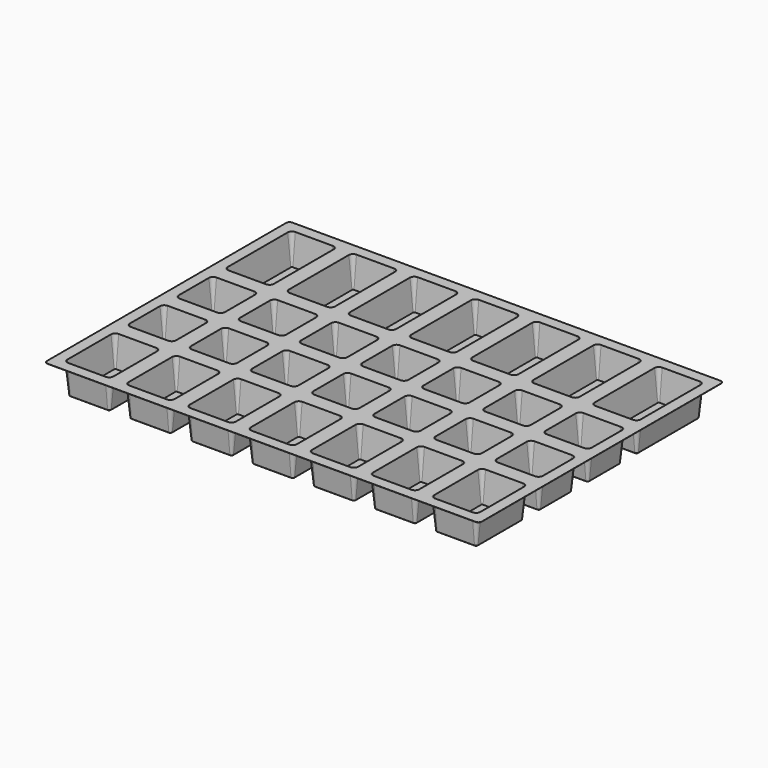
from build123d import *

# Parameters (mm, degrees)
F1_W     = 256
F1_H     = 180
F2_DEPTH = 0.1
F3_DEPTH = 25
F4_DEPTH = 18
F4_TAPER = 6
F5_T     = 0.5
F5_2_T   = -0.5
F5_3_T   = 0.5
F5_4_T   = 0.5
F5_5_T   = -0.5
F5_6_T   = 0.5
F5_7_T   = 0.5
F5_8_T   = -0.5
F5_9_T   = -0.5
F5_10_T  = 0.5
F5_11_T  = 0.5
F5_12_T  = -0.5
F5_13_T  = -0.5
F5_14_T  = 0.5
F5_15_T  = 0.5
F5_16_T  = -0.5
F5_17_T  = -0.5
F5_18_T  = 0.5
F5_19_T  = -0.5
F5_20_T  = 0.5
F5_21_T  = 0.5
F5_22_T  = -0.5
F5_23_T  = 0.5
F5_24_T  = -0.5
F5_25_T  = -0.5
F5_26_T  = 0.5
F5_27_T  = -0.5
F5_28_T  = 0.5
F6_R     = 2
F7_R     = 0.5
F7_2_R   = 0.5
F7_3_R   = 0.5
F7_4_R   = 0.5
F7_5_R   = 0.5
F7_6_R   = 0.5
F7_7_R   = 0.5
F7_8_R   = 0.5
F7_9_R   = 0.5
F7_10_R  = 0.5
F7_11_R  = 0.5
F7_12_R  = 0.5
F7_13_R  = 0.5
F7_14_R  = 0.5
F7_15_R  = 0.5
F7_16_R  = 0.5
F7_17_R  = 0.5
F7_18_R  = 0.5
F7_19_R  = 0.5
F7_20_R  = 0.5
F7_21_R  = 0.5
F7_22_R  = 0.5
F7_23_R  = 0.5
F7_24_R  = 0.5
F7_25_R  = 0.5
F7_26_R  = 0.5
F7_27_R  = 0.5
F7_28_R  = 0.5


# Not quite as in the source:
# - a shell that OpenCascade refuses in one call is made with other operations: the cavity is built on its own and cut out


with BuildPart() as f2:
    # F1 (on Top) → F2 (new body)
    with BuildSketch(Plane.XY):
        with Locations((132.6459416151, -90)):
            Rectangle(F1_W, F1_H)
    extrude(amount=-F2_DEPTH)

    # F0 (on Top) → F3 (cut)
    with BuildSketch(Plane.XY):
        with BuildLine():
            ThreePointArc((121.6459416151, -6), (119.5246212715, -6.8786796564), (118.6459416151, -9))
            Line((118.6459416151, -9), (118.6459416151, -53))
            ThreePointArc((118.6459416151, -53), (119.5246212715, -55.1213203436), (121.6459416151, -56))
            Line((121.6459416151, -56), (143.6459416151, -56))
            ThreePointArc((143.6459416151, -56), (145.7672619587, -55.1213203436), (146.6459416151, -53))
            Line((146.6459416151, -53), (146.6459416151, -9))
            ThreePointArc((146.6459416151, -9), (145.7672619587, -6.8786796564), (143.6459416151, -6))
            Line((143.6459416151, -6), (121.6459416151, -6))
        make_face()
        with BuildLine():
            Line((146.6459416151, -89), (146.6459416151, -67))
            ThreePointArc((146.6459416151, -67), (145.7672619587, -64.8786796564), (143.6459416151, -64))
            Line((143.6459416151, -64), (121.6459416151, -64))
            ThreePointArc((121.6459416151, -64), (119.5246212715, -64.8786796564), (118.6459416151, -67))
            Line((118.6459416151, -67), (118.6459416151, -89))
            ThreePointArc((118.6459416151, -89), (119.5246212715, -91.1213203436), (121.6459416151, -92))
            Line((121.6459416151, -92), (143.6459416151, -92))
            ThreePointArc((143.6459416151, -92), (145.7672619587, -91.1213203436), (146.6459416151, -89))
        make_face()
        with BuildLine():
            Line((146.6459416151, -125), (146.6459416151, -103))
            ThreePointArc((146.6459416151, -103), (145.7672619587, -100.8786796564), (143.6459416151, -100))
            Line((143.6459416151, -100), (121.6459416151, -100))
            ThreePointArc((121.6459416151, -100), (119.5246212715, -100.8786796564), (118.6459416151, -103))
            Line((118.6459416151, -103), (118.6459416151, -125))
            ThreePointArc((118.6459416151, -125), (119.5246212715, -127.1213203436), (121.6459416151, -128))
            Line((121.6459416151, -128), (143.6459416151, -128))
            ThreePointArc((143.6459416151, -128), (145.7672619587, -127.1213203436), (146.6459416151, -125))
        make_face()
        with BuildLine():
            Line((146.6459416151, -171), (146.6459416151, -139))
            ThreePointArc((146.6459416151, -139), (145.7672619587, -136.8786796564), (143.6459416151, -136))
            Line((143.6459416151, -136), (121.6459416151, -136))
            ThreePointArc((121.6459416151, -136), (119.5246212715, -136.8786796564), (118.6459416151, -139))
            Line((118.6459416151, -139), (118.6459416151, -171))
            ThreePointArc((118.6459416151, -171), (119.5246212715, -173.1213203436), (121.6459416151, -174))
            Line((121.6459416151, -174), (143.6459416151, -174))
            ThreePointArc((143.6459416151, -174), (145.7672619587, -173.1213203436), (146.6459416151, -171))
        make_face()
        with BuildLine():
            ThreePointArc((157.6459416151, -6), (155.5246212715, -6.8786796564), (154.6459416151, -9))
            Line((154.6459416151, -9), (154.6459416151, -53))
            ThreePointArc((154.6459416151, -53), (155.5246212715, -55.1213203436), (157.6459416151, -56))
            Line((157.6459416151, -56), (179.6459416151, -56))
            ThreePointArc((179.6459416151, -56), (181.7672619587, -55.1213203436), (182.6459416151, -53))
            Line((182.6459416151, -53), (182.6459416151, -9))
            ThreePointArc((182.6459416151, -9), (181.7672619587, -6.8786796564), (179.6459416151, -6))
            Line((179.6459416151, -6), (157.6459416151, -6))
        make_face()
        with BuildLine():
            Line((182.6459416151, -89), (182.6459416151, -67))
            ThreePointArc((182.6459416151, -67), (181.7672619587, -64.8786796564), (179.6459416151, -64))
            Line((179.6459416151, -64), (157.6459416151, -64))
            ThreePointArc((157.6459416151, -64), (155.5246212715, -64.8786796564), (154.6459416151, -67))
            Line((154.6459416151, -67), (154.6459416151, -89))
            ThreePointArc((154.6459416151, -89), (155.5246212715, -91.1213203436), (157.6459416151, -92))
            Line((157.6459416151, -92), (179.6459416151, -92))
            ThreePointArc((179.6459416151, -92), (181.7672619587, -91.1213203436), (182.6459416151, -89))
        make_face()
        with BuildLine():
            ThreePointArc((157.6459416151, -136), (155.5246212715, -136.8786796564), (154.6459416151, -139))
            Line((154.6459416151, -139), (154.6459416151, -171))
            ThreePointArc((154.6459416151, -171), (155.5246212715, -173.1213203436), (157.6459416151, -174))
            Line((157.6459416151, -174), (179.6459416151, -174))
            ThreePointArc((179.6459416151, -174), (181.7672619587, -173.1213203436), (182.6459416151, -171))
            Line((182.6459416151, -171), (182.6459416151, -139))
            ThreePointArc((182.6459416151, -139), (181.7672619587, -136.8786796564), (179.6459416151, -136))
            Line((179.6459416151, -136), (157.6459416151, -136))
        make_face()
        with BuildLine():
            Line((182.6459416151, -125), (182.6459416151, -103))
            ThreePointArc((182.6459416151, -103), (181.7672619587, -100.8786796564), (179.6459416151, -100))
            Line((179.6459416151, -100), (157.6459416151, -100))
            ThreePointArc((157.6459416151, -100), (155.5246212715, -100.8786796564), (154.6459416151, -103))
            Line((154.6459416151, -103), (154.6459416151, -125))
            ThreePointArc((154.6459416151, -125), (155.5246212715, -127.1213203436), (157.6459416151, -128))
            Line((157.6459416151, -128), (179.6459416151, -128))
            ThreePointArc((179.6459416151, -128), (181.7672619587, -127.1213203436), (182.6459416151, -125))
        make_face()
        with BuildLine():
            ThreePointArc((193.6459416151, -6), (191.5246212715, -6.8786796564), (190.6459416151, -9))
            Line((190.6459416151, -9), (190.6459416151, -53))
            ThreePointArc((190.6459416151, -53), (191.5246212715, -55.1213203436), (193.6459416151, -56))
            Line((193.6459416151, -56), (215.6459416151, -56))
            ThreePointArc((215.6459416151, -56), (217.7672619587, -55.1213203436), (218.6459416151, -53))
            Line((218.6459416151, -53), (218.6459416151, -9))
            ThreePointArc((218.6459416151, -9), (217.7672619587, -6.8786796564), (215.6459416151, -6))
            Line((215.6459416151, -6), (193.6459416151, -6))
        make_face()
        with BuildLine():
            Line((218.6459416151, -89), (218.6459416151, -67))
            ThreePointArc((218.6459416151, -67), (217.7672619587, -64.8786796564), (215.6459416151, -64))
            Line((215.6459416151, -64), (193.6459416151, -64))
            ThreePointArc((193.6459416151, -64), (191.5246212715, -64.8786796564), (190.6459416151, -67))
            Line((190.6459416151, -67), (190.6459416151, -89))
            ThreePointArc((190.6459416151, -89), (191.5246212715, -91.1213203436), (193.6459416151, -92))
            Line((193.6459416151, -92), (215.6459416151, -92))
            ThreePointArc((215.6459416151, -92), (217.7672619587, -91.1213203436), (218.6459416151, -89))
        make_face()
        with BuildLine():
            ThreePointArc((193.6459416151, -136), (191.5246212715, -136.8786796564), (190.6459416151, -139))
            Line((190.6459416151, -139), (190.6459416151, -171))
            ThreePointArc((190.6459416151, -171), (191.5246212715, -173.1213203436), (193.6459416151, -174))
            Line((193.6459416151, -174), (215.6459416151, -174))
            ThreePointArc((215.6459416151, -174), (217.7672619587, -173.1213203436), (218.6459416151, -171))
            Line((218.6459416151, -171), (218.6459416151, -139))
            ThreePointArc((218.6459416151, -139), (217.7672619587, -136.8786796564), (215.6459416151, -136))
            Line((215.6459416151, -136), (193.6459416151, -136))
        make_face()
        with BuildLine():
            Line((218.6459416151, -125), (218.6459416151, -103))
            ThreePointArc((218.6459416151, -103), (217.7672619587, -100.8786796564), (215.6459416151, -100))
            Line((215.6459416151, -100), (193.6459416151, -100))
            ThreePointArc((193.6459416151, -100), (191.5246212715, -100.8786796564), (190.6459416151, -103))
            Line((190.6459416151, -103), (190.6459416151, -125))
            ThreePointArc((190.6459416151, -125), (191.5246212715, -127.1213203436), (193.6459416151, -128))
            Line((193.6459416151, -128), (215.6459416151, -128))
            ThreePointArc((215.6459416151, -128), (217.7672619587, -127.1213203436), (218.6459416151, -125))
        make_face()
        with BuildLine():
            ThreePointArc((229.6459416151, -6), (227.5246212715, -6.8786796564), (226.6459416151, -9))
            Line((226.6459416151, -9), (226.6459416151, -53))
            ThreePointArc((226.6459416151, -53), (227.5246212715, -55.1213203436), (229.6459416151, -56))
            Line((229.6459416151, -56), (251.6459416151, -56))
            ThreePointArc((251.6459416151, -56), (253.7672619587, -55.1213203436), (254.6459416151, -53))
            Line((254.6459416151, -53), (254.6459416151, -9))
            ThreePointArc((254.6459416151, -9), (253.7672619587, -6.8786796564), (251.6459416151, -6))
            Line((251.6459416151, -6), (229.6459416151, -6))
        make_face()
        with BuildLine():
            Line((254.6459416151, -89), (254.6459416151, -67))
            ThreePointArc((254.6459416151, -67), (253.7672619587, -64.8786796564), (251.6459416151, -64))
            Line((251.6459416151, -64), (229.6459416151, -64))
            ThreePointArc((229.6459416151, -64), (227.5246212715, -64.8786796564), (226.6459416151, -67))
            Line((226.6459416151, -67), (226.6459416151, -89))
            ThreePointArc((226.6459416151, -89), (227.5246212715, -91.1213203436), (229.6459416151, -92))
            Line((229.6459416151, -92), (251.6459416151, -92))
            ThreePointArc((251.6459416151, -92), (253.7672619587, -91.1213203436), (254.6459416151, -89))
        make_face()
        with BuildLine():
            ThreePointArc((229.6459416151, -136), (227.5246212715, -136.8786796564), (226.6459416151, -139))
            Line((226.6459416151, -139), (226.6459416151, -171))
            ThreePointArc((226.6459416151, -171), (227.5246212715, -173.1213203436), (229.6459416151, -174))
            Line((229.6459416151, -174), (251.6459416151, -174))
            ThreePointArc((251.6459416151, -174), (253.7672619587, -173.1213203436), (254.6459416151, -171))
            Line((254.6459416151, -171), (254.6459416151, -139))
            ThreePointArc((254.6459416151, -139), (253.7672619587, -136.8786796564), (251.6459416151, -136))
            Line((251.6459416151, -136), (229.6459416151, -136))
        make_face()
        with BuildLine():
            Line((254.6459416151, -125), (254.6459416151, -103))
            ThreePointArc((254.6459416151, -103), (253.7672619587, -100.8786796564), (251.6459416151, -100))
            Line((251.6459416151, -100), (229.6459416151, -100))
            ThreePointArc((229.6459416151, -100), (227.5246212715, -100.8786796564), (226.6459416151, -103))
            Line((226.6459416151, -103), (226.6459416151, -125))
            ThreePointArc((226.6459416151, -125), (227.5246212715, -127.1213203436), (229.6459416151, -128))
            Line((229.6459416151, -128), (251.6459416151, -128))
            ThreePointArc((251.6459416151, -128), (253.7672619587, -127.1213203436), (254.6459416151, -125))
        make_face()
        with BuildLine():
            Line((85.6459416151, -92), (107.6459416151, -92))
            ThreePointArc((107.6459416151, -92), (109.7672619587, -91.1213203436), (110.6459416151, -89))
            Line((110.6459416151, -89), (110.6459416151, -67))
            ThreePointArc((110.6459416151, -67), (109.7672619587, -64.8786796564), (107.6459416151, -64))
            Line((107.6459416151, -64), (85.6459416151, -64))
            ThreePointArc((85.6459416151, -64), (83.5246212715, -64.8786796564), (82.6459416151, -67))
            Line((82.6459416151, -67), (82.6459416151, -89))
            ThreePointArc((82.6459416151, -89), (83.5246212715, -91.1213203436), (85.6459416151, -92))
        make_face()
        with BuildLine():
            Line((85.6459416151, -128), (107.6459416151, -128))
            ThreePointArc((107.6459416151, -128), (109.7672619587, -127.1213203436), (110.6459416151, -125))
            Line((110.6459416151, -125), (110.6459416151, -103))
            ThreePointArc((110.6459416151, -103), (109.7672619587, -100.8786796564), (107.6459416151, -100))
            Line((107.6459416151, -100), (85.6459416151, -100))
            ThreePointArc((85.6459416151, -100), (83.5246212715, -100.8786796564), (82.6459416151, -103))
            Line((82.6459416151, -103), (82.6459416151, -125))
            ThreePointArc((82.6459416151, -125), (83.5246212715, -127.1213203436), (85.6459416151, -128))
        make_face()
        with BuildLine():
            ThreePointArc((85.6459416151, -136), (83.5246212715, -136.8786796564), (82.6459416151, -139))
            Line((82.6459416151, -139), (82.6459416151, -171))
            ThreePointArc((82.6459416151, -171), (83.5246212715, -173.1213203436), (85.6459416151, -174))
            Line((85.6459416151, -174), (107.6459416151, -174))
            ThreePointArc((107.6459416151, -174), (109.7672619587, -173.1213203436), (110.6459416151, -171))
            Line((110.6459416151, -171), (110.6459416151, -139))
            ThreePointArc((110.6459416151, -139), (109.7672619587, -136.8786796564), (107.6459416151, -136))
            Line((107.6459416151, -136), (85.6459416151, -136))
        make_face()
        with BuildLine():
            Line((110.6459416151, -53), (110.6459416151, -9))
            ThreePointArc((110.6459416151, -9), (109.7672619587, -6.8786796564), (107.6459416151, -6))
            Line((107.6459416151, -6), (85.6459416151, -6))
            ThreePointArc((85.6459416151, -6), (83.5246212715, -6.8786796564), (82.6459416151, -9))
            Line((82.6459416151, -9), (82.6459416151, -53))
            ThreePointArc((82.6459416151, -53), (83.5246212715, -55.1213203436), (85.6459416151, -56))
            Line((85.6459416151, -56), (107.6459416151, -56))
            ThreePointArc((107.6459416151, -56), (109.7672619587, -55.1213203436), (110.6459416151, -53))
        make_face()
        with BuildLine():
            Line((49.6459416151, -92), (71.6459416151, -92))
            ThreePointArc((71.6459416151, -92), (73.7672619587, -91.1213203436), (74.6459416151, -89))
            Line((74.6459416151, -89), (74.6459416151, -67))
            ThreePointArc((74.6459416151, -67), (73.7672619587, -64.8786796564), (71.6459416151, -64))
            Line((71.6459416151, -64), (49.6459416151, -64))
            ThreePointArc((49.6459416151, -64), (47.5246212715, -64.8786796564), (46.6459416151, -67))
            Line((46.6459416151, -67), (46.6459416151, -89))
            ThreePointArc((46.6459416151, -89), (47.5246212715, -91.1213203436), (49.6459416151, -92))
        make_face()
        with BuildLine():
            Line((49.6459416151, -128), (71.6459416151, -128))
            ThreePointArc((71.6459416151, -128), (73.7672619587, -127.1213203436), (74.6459416151, -125))
            Line((74.6459416151, -125), (74.6459416151, -103))
            ThreePointArc((74.6459416151, -103), (73.7672619587, -100.8786796564), (71.6459416151, -100))
            Line((71.6459416151, -100), (49.6459416151, -100))
            ThreePointArc((49.6459416151, -100), (47.5246212715, -100.8786796564), (46.6459416151, -103))
            Line((46.6459416151, -103), (46.6459416151, -125))
            ThreePointArc((46.6459416151, -125), (47.5246212715, -127.1213203436), (49.6459416151, -128))
        make_face()
        with BuildLine():
            ThreePointArc((49.6459416151, -136), (47.5246212715, -136.8786796564), (46.6459416151, -139))
            Line((46.6459416151, -139), (46.6459416151, -171))
            ThreePointArc((46.6459416151, -171), (47.5246212715, -173.1213203436), (49.6459416151, -174))
            Line((49.6459416151, -174), (71.6459416151, -174))
            ThreePointArc((71.6459416151, -174), (73.7672619587, -173.1213203436), (74.6459416151, -171))
            Line((74.6459416151, -171), (74.6459416151, -139))
            ThreePointArc((74.6459416151, -139), (73.7672619587, -136.8786796564), (71.6459416151, -136))
            Line((71.6459416151, -136), (49.6459416151, -136))
        make_face()
        with BuildLine():
            Line((74.6459416151, -53), (74.6459416151, -9))
            ThreePointArc((74.6459416151, -9), (73.7672619587, -6.8786796564), (71.6459416151, -6))
            Line((71.6459416151, -6), (49.6459416151, -6))
            ThreePointArc((49.6459416151, -6), (47.5246212715, -6.8786796564), (46.6459416151, -9))
            Line((46.6459416151, -9), (46.6459416151, -53))
            ThreePointArc((46.6459416151, -53), (47.5246212715, -55.1213203436), (49.6459416151, -56))
            Line((49.6459416151, -56), (71.6459416151, -56))
            ThreePointArc((71.6459416151, -56), (73.7672619587, -55.1213203436), (74.6459416151, -53))
        make_face()
        with BuildLine():
            Line((13.6459416151, -92), (35.6459416151, -92))
            ThreePointArc((35.6459416151, -92), (37.7672619587, -91.1213203436), (38.6459416151, -89))
            Line((38.6459416151, -89), (38.6459416151, -67))
            ThreePointArc((38.6459416151, -67), (37.7672619587, -64.8786796564), (35.6459416151, -64))
            Line((35.6459416151, -64), (13.6459416151, -64))
            ThreePointArc((13.6459416151, -64), (11.5246212715, -64.8786796564), (10.6459416151, -67))
            Line((10.6459416151, -67), (10.6459416151, -89))
            ThreePointArc((10.6459416151, -89), (11.5246212715, -91.1213203436), (13.6459416151, -92))
        make_face()
        with BuildLine():
            Line((13.6459416151, -128), (35.6459416151, -128))
            ThreePointArc((35.6459416151, -128), (37.7672619587, -127.1213203436), (38.6459416151, -125))
            Line((38.6459416151, -125), (38.6459416151, -103))
            ThreePointArc((38.6459416151, -103), (37.7672619587, -100.8786796564), (35.6459416151, -100))
            Line((35.6459416151, -100), (13.6459416151, -100))
            ThreePointArc((13.6459416151, -100), (11.5246212715, -100.8786796564), (10.6459416151, -103))
            Line((10.6459416151, -103), (10.6459416151, -125))
            ThreePointArc((10.6459416151, -125), (11.5246212715, -127.1213203436), (13.6459416151, -128))
        make_face()
        with BuildLine():
            ThreePointArc((13.6459416151, -136), (11.5246212715, -136.8786796564), (10.6459416151, -139))
            Line((10.6459416151, -139), (10.6459416151, -171))
            ThreePointArc((10.6459416151, -171), (11.5246212715, -173.1213203436), (13.6459416151, -174))
            Line((13.6459416151, -174), (35.6459416151, -174))
            ThreePointArc((35.6459416151, -174), (37.7672619587, -173.1213203436), (38.6459416151, -171))
            Line((38.6459416151, -171), (38.6459416151, -139))
            ThreePointArc((38.6459416151, -139), (37.7672619587, -136.8786796564), (35.6459416151, -136))
            Line((35.6459416151, -136), (13.6459416151, -136))
        make_face()
        with BuildLine():
            Line((38.6459416151, -53), (38.6459416151, -9))
            ThreePointArc((38.6459416151, -9), (37.7672619587, -6.8786796564), (35.6459416151, -6))
            Line((35.6459416151, -6), (13.6459416151, -6))
            ThreePointArc((13.6459416151, -6), (11.5246212715, -6.8786796564), (10.6459416151, -9))
            Line((10.6459416151, -9), (10.6459416151, -53))
            ThreePointArc((10.6459416151, -53), (11.5246212715, -55.1213203436), (13.6459416151, -56))
            Line((13.6459416151, -56), (35.6459416151, -56))
            ThreePointArc((35.6459416151, -56), (37.7672619587, -55.1213203436), (38.6459416151, -53))
        make_face()
    extrude(amount=-F3_DEPTH, mode=Mode.SUBTRACT)

    # F6
    f6_edges = [f2.edges().sort_by_distance(p)[0] for p in [
        (4.645942, -180, -0.05),
        (260.645942, -180, -0.05),
        (260.645942, 0, -0.05),
        (4.645942, 0, -0.05),
    ]]
    fillet(f6_edges, radius=F6_R)


with BuildPart() as f4:
    # F0 (on Top) → F4 (new body)
    with BuildSketch(Plane.XY):
        with BuildLine():
            ThreePointArc((121.6459416151, -6), (119.5246212715, -6.8786796564), (118.6459416151, -9))
            Line((118.6459416151, -9), (118.6459416151, -53))
            ThreePointArc((118.6459416151, -53), (119.5246212715, -55.1213203436), (121.6459416151, -56))
            Line((121.6459416151, -56), (143.6459416151, -56))
            ThreePointArc((143.6459416151, -56), (145.7672619587, -55.1213203436), (146.6459416151, -53))
            Line((146.6459416151, -53), (146.6459416151, -9))
            ThreePointArc((146.6459416151, -9), (145.7672619587, -6.8786796564), (143.6459416151, -6))
            Line((143.6459416151, -6), (121.6459416151, -6))
        make_face()
    extrude(amount=-F4_DEPTH, taper=F4_TAPER)

    # F5: shell of thickness 0.5, made by hand


with BuildPart() as f4b:
    # F0 (on Top) → F4, piece 2 (new body)
    with BuildSketch(Plane.XY):
        with BuildLine():
            Line((146.6459416151, -89), (146.6459416151, -67))
            ThreePointArc((146.6459416151, -67), (145.7672619587, -64.8786796564), (143.6459416151, -64))
            Line((143.6459416151, -64), (121.6459416151, -64))
            ThreePointArc((121.6459416151, -64), (119.5246212715, -64.8786796564), (118.6459416151, -67))
            Line((118.6459416151, -67), (118.6459416151, -89))
            ThreePointArc((118.6459416151, -89), (119.5246212715, -91.1213203436), (121.6459416151, -92))
            Line((121.6459416151, -92), (143.6459416151, -92))
            ThreePointArc((143.6459416151, -92), (145.7672619587, -91.1213203436), (146.6459416151, -89))
        make_face()
    extrude(amount=-F4_DEPTH, taper=F4_TAPER)

    # F5#2
    f5_2_openings = [f4b.faces().sort_by_distance(p)[0] for p in [
        (132.645942, -78, 0),
    ]]
    offset(amount=F5_2_T, openings=f5_2_openings)

    # F7#2
    f7_2_edges = [f4b.edges().sort_by_distance(p)[0] for p in [
        (144.429503, -89.783562, -18),
        (144.754065, -78, -18),
        (144.429503, -66.216438, -18),
        (132.645942, -65.891876, -18),
        (120.86238, -66.216438, -18),
        (120.537818, -78, -18),
        (120.86238, -89.783562, -18),
        (132.645942, -90.108124, -18),
    ]]
    fillet(f7_2_edges, radius=F7_2_R)


with BuildPart() as f4c:
    # F0 (on Top) → F4, piece 3 (new body)
    with BuildSketch(Plane.XY):
        with BuildLine():
            Line((146.6459416151, -125), (146.6459416151, -103))
            ThreePointArc((146.6459416151, -103), (145.7672619587, -100.8786796564), (143.6459416151, -100))
            Line((143.6459416151, -100), (121.6459416151, -100))
            ThreePointArc((121.6459416151, -100), (119.5246212715, -100.8786796564), (118.6459416151, -103))
            Line((118.6459416151, -103), (118.6459416151, -125))
            ThreePointArc((118.6459416151, -125), (119.5246212715, -127.1213203436), (121.6459416151, -128))
            Line((121.6459416151, -128), (143.6459416151, -128))
            ThreePointArc((143.6459416151, -128), (145.7672619587, -127.1213203436), (146.6459416151, -125))
        make_face()
    extrude(amount=-F4_DEPTH, taper=F4_TAPER)

    # F5#3: shell of thickness 0.5, made by hand


with BuildPart() as f4d:
    # F0 (on Top) → F4, piece 4 (new body)
    with BuildSketch(Plane.XY):
        with BuildLine():
            Line((146.6459416151, -171), (146.6459416151, -139))
            ThreePointArc((146.6459416151, -139), (145.7672619587, -136.8786796564), (143.6459416151, -136))
            Line((143.6459416151, -136), (121.6459416151, -136))
            ThreePointArc((121.6459416151, -136), (119.5246212715, -136.8786796564), (118.6459416151, -139))
            Line((118.6459416151, -139), (118.6459416151, -171))
            ThreePointArc((118.6459416151, -171), (119.5246212715, -173.1213203436), (121.6459416151, -174))
            Line((121.6459416151, -174), (143.6459416151, -174))
            ThreePointArc((143.6459416151, -174), (145.7672619587, -173.1213203436), (146.6459416151, -171))
        make_face()
    extrude(amount=-F4_DEPTH, taper=F4_TAPER)

    # F5#4: shell of thickness 0.5, made by hand


with BuildPart() as f4e:
    # F0 (on Top) → F4, piece 5 (new body)
    with BuildSketch(Plane.XY):
        with BuildLine():
            ThreePointArc((157.6459416151, -6), (155.5246212715, -6.8786796564), (154.6459416151, -9))
            Line((154.6459416151, -9), (154.6459416151, -53))
            ThreePointArc((154.6459416151, -53), (155.5246212715, -55.1213203436), (157.6459416151, -56))
            Line((157.6459416151, -56), (179.6459416151, -56))
            ThreePointArc((179.6459416151, -56), (181.7672619587, -55.1213203436), (182.6459416151, -53))
            Line((182.6459416151, -53), (182.6459416151, -9))
            ThreePointArc((182.6459416151, -9), (181.7672619587, -6.8786796564), (179.6459416151, -6))
            Line((179.6459416151, -6), (157.6459416151, -6))
        make_face()
    extrude(amount=-F4_DEPTH, taper=F4_TAPER)

    # F5#13
    f5_13_openings = [f4e.faces().sort_by_distance(p)[0] for p in [
        (168.645942, -31, 0),
    ]]
    offset(amount=F5_13_T, openings=f5_13_openings)

    # F7#17
    f7_17_edges = [f4e.edges().sort_by_distance(p)[0] for p in [
        (156.86238, -8.216438, -18),
        (156.537818, -31, -18),
        (156.86238, -53.783562, -18),
        (168.645942, -54.108124, -18),
        (180.429503, -53.783562, -18),
        (180.754065, -31, -18),
        (180.429503, -8.216438, -18),
        (168.645942, -7.891876, -18),
    ]]
    fillet(f7_17_edges, radius=F7_17_R)


with BuildPart() as f4f:
    # F0 (on Top) → F4, piece 6 (new body)
    with BuildSketch(Plane.XY):
        with BuildLine():
            Line((182.6459416151, -89), (182.6459416151, -67))
            ThreePointArc((182.6459416151, -67), (181.7672619587, -64.8786796564), (179.6459416151, -64))
            Line((179.6459416151, -64), (157.6459416151, -64))
            ThreePointArc((157.6459416151, -64), (155.5246212715, -64.8786796564), (154.6459416151, -67))
            Line((154.6459416151, -67), (154.6459416151, -89))
            ThreePointArc((154.6459416151, -89), (155.5246212715, -91.1213203436), (157.6459416151, -92))
            Line((157.6459416151, -92), (179.6459416151, -92))
            ThreePointArc((179.6459416151, -92), (181.7672619587, -91.1213203436), (182.6459416151, -89))
        make_face()
    extrude(amount=-F4_DEPTH, taper=F4_TAPER)

    # F5#14: shell of thickness 0.5, made by hand


with BuildPart() as f4g:
    # F0 (on Top) → F4, piece 7 (new body)
    with BuildSketch(Plane.XY):
        with BuildLine():
            ThreePointArc((157.6459416151, -136), (155.5246212715, -136.8786796564), (154.6459416151, -139))
            Line((154.6459416151, -139), (154.6459416151, -171))
            ThreePointArc((154.6459416151, -171), (155.5246212715, -173.1213203436), (157.6459416151, -174))
            Line((157.6459416151, -174), (179.6459416151, -174))
            ThreePointArc((179.6459416151, -174), (181.7672619587, -173.1213203436), (182.6459416151, -171))
            Line((182.6459416151, -171), (182.6459416151, -139))
            ThreePointArc((182.6459416151, -139), (181.7672619587, -136.8786796564), (179.6459416151, -136))
            Line((179.6459416151, -136), (157.6459416151, -136))
        make_face()
    extrude(amount=-F4_DEPTH, taper=F4_TAPER)

    # F5#16
    f5_16_openings = [f4g.faces().sort_by_distance(p)[0] for p in [
        (168.645942, -155, 0),
    ]]
    offset(amount=F5_16_T, openings=f5_16_openings)

    # F7#20
    f7_20_edges = [f4g.edges().sort_by_distance(p)[0] for p in [
        (180.429503, -138.216438, -18),
        (168.645942, -137.891876, -18),
        (156.86238, -138.216438, -18),
        (156.537818, -155, -18),
        (156.86238, -171.783562, -18),
        (168.645942, -172.108124, -18),
        (180.429503, -171.783562, -18),
        (180.754065, -155, -18),
    ]]
    fillet(f7_20_edges, radius=F7_20_R)


with BuildPart() as f4h:
    # F0 (on Top) → F4, piece 8 (new body)
    with BuildSketch(Plane.XY):
        with BuildLine():
            Line((182.6459416151, -125), (182.6459416151, -103))
            ThreePointArc((182.6459416151, -103), (181.7672619587, -100.8786796564), (179.6459416151, -100))
            Line((179.6459416151, -100), (157.6459416151, -100))
            ThreePointArc((157.6459416151, -100), (155.5246212715, -100.8786796564), (154.6459416151, -103))
            Line((154.6459416151, -103), (154.6459416151, -125))
            ThreePointArc((154.6459416151, -125), (155.5246212715, -127.1213203436), (157.6459416151, -128))
            Line((157.6459416151, -128), (179.6459416151, -128))
            ThreePointArc((179.6459416151, -128), (181.7672619587, -127.1213203436), (182.6459416151, -125))
        make_face()
    extrude(amount=-F4_DEPTH, taper=F4_TAPER)

    # F5#15: shell of thickness 0.5, made by hand


with BuildPart() as f4i:
    # F0 (on Top) → F4, piece 9 (new body)
    with BuildSketch(Plane.XY):
        with BuildLine():
            ThreePointArc((193.6459416151, -6), (191.5246212715, -6.8786796564), (190.6459416151, -9))
            Line((190.6459416151, -9), (190.6459416151, -53))
            ThreePointArc((190.6459416151, -53), (191.5246212715, -55.1213203436), (193.6459416151, -56))
            Line((193.6459416151, -56), (215.6459416151, -56))
            ThreePointArc((215.6459416151, -56), (217.7672619587, -55.1213203436), (218.6459416151, -53))
            Line((218.6459416151, -53), (218.6459416151, -9))
            ThreePointArc((218.6459416151, -9), (217.7672619587, -6.8786796564), (215.6459416151, -6))
            Line((215.6459416151, -6), (193.6459416151, -6))
        make_face()
    extrude(amount=-F4_DEPTH, taper=F4_TAPER)

    # F5#12
    f5_12_openings = [f4i.faces().sort_by_distance(p)[0] for p in [
        (204.645942, -31, 0),
    ]]
    offset(amount=F5_12_T, openings=f5_12_openings)

    # F7#24
    f7_24_edges = [f4i.edges().sort_by_distance(p)[0] for p in [
        (192.86238, -8.216438, -18),
        (192.537818, -31, -18),
        (192.86238, -53.783562, -18),
        (204.645942, -54.108124, -18),
        (216.429503, -53.783562, -18),
        (216.754065, -31, -18),
        (216.429503, -8.216438, -18),
        (204.645942, -7.891876, -18),
    ]]
    fillet(f7_24_edges, radius=F7_24_R)


with BuildPart() as f4j:
    # F0 (on Top) → F4, piece 10 (new body)
    with BuildSketch(Plane.XY):
        with BuildLine():
            Line((218.6459416151, -89), (218.6459416151, -67))
            ThreePointArc((218.6459416151, -67), (217.7672619587, -64.8786796564), (215.6459416151, -64))
            Line((215.6459416151, -64), (193.6459416151, -64))
            ThreePointArc((193.6459416151, -64), (191.5246212715, -64.8786796564), (190.6459416151, -67))
            Line((190.6459416151, -67), (190.6459416151, -89))
            ThreePointArc((190.6459416151, -89), (191.5246212715, -91.1213203436), (193.6459416151, -92))
            Line((193.6459416151, -92), (215.6459416151, -92))
            ThreePointArc((215.6459416151, -92), (217.7672619587, -91.1213203436), (218.6459416151, -89))
        make_face()
    extrude(amount=-F4_DEPTH, taper=F4_TAPER)

    # F5#11: shell of thickness 0.5, made by hand


with BuildPart() as f4k:
    # F0 (on Top) → F4, piece 11 (new body)
    with BuildSketch(Plane.XY):
        with BuildLine():
            ThreePointArc((193.6459416151, -136), (191.5246212715, -136.8786796564), (190.6459416151, -139))
            Line((190.6459416151, -139), (190.6459416151, -171))
            ThreePointArc((190.6459416151, -171), (191.5246212715, -173.1213203436), (193.6459416151, -174))
            Line((193.6459416151, -174), (215.6459416151, -174))
            ThreePointArc((215.6459416151, -174), (217.7672619587, -173.1213203436), (218.6459416151, -171))
            Line((218.6459416151, -171), (218.6459416151, -139))
            ThreePointArc((218.6459416151, -139), (217.7672619587, -136.8786796564), (215.6459416151, -136))
            Line((215.6459416151, -136), (193.6459416151, -136))
        make_face()
    extrude(amount=-F4_DEPTH, taper=F4_TAPER)

    # F5#9
    f5_9_openings = [f4k.faces().sort_by_distance(p)[0] for p in [
        (204.645942, -155, 0),
    ]]
    offset(amount=F5_9_T, openings=f5_9_openings)

    # F7#21
    f7_21_edges = [f4k.edges().sort_by_distance(p)[0] for p in [
        (216.429503, -138.216438, -18),
        (204.645942, -137.891876, -18),
        (192.86238, -138.216438, -18),
        (192.537818, -155, -18),
        (192.86238, -171.783562, -18),
        (204.645942, -172.108124, -18),
        (216.429503, -171.783562, -18),
        (216.754065, -155, -18),
    ]]
    fillet(f7_21_edges, radius=F7_21_R)


with BuildPart() as f4l:
    # F0 (on Top) → F4, piece 12 (new body)
    with BuildSketch(Plane.XY):
        with BuildLine():
            Line((218.6459416151, -125), (218.6459416151, -103))
            ThreePointArc((218.6459416151, -103), (217.7672619587, -100.8786796564), (215.6459416151, -100))
            Line((215.6459416151, -100), (193.6459416151, -100))
            ThreePointArc((193.6459416151, -100), (191.5246212715, -100.8786796564), (190.6459416151, -103))
            Line((190.6459416151, -103), (190.6459416151, -125))
            ThreePointArc((190.6459416151, -125), (191.5246212715, -127.1213203436), (193.6459416151, -128))
            Line((193.6459416151, -128), (215.6459416151, -128))
            ThreePointArc((215.6459416151, -128), (217.7672619587, -127.1213203436), (218.6459416151, -125))
        make_face()
    extrude(amount=-F4_DEPTH, taper=F4_TAPER)

    # F5#10: shell of thickness 0.5, made by hand


with BuildPart() as f4m:
    # F0 (on Top) → F4, piece 13 (new body)
    with BuildSketch(Plane.XY):
        with BuildLine():
            ThreePointArc((229.6459416151, -6), (227.5246212715, -6.8786796564), (226.6459416151, -9))
            Line((226.6459416151, -9), (226.6459416151, -53))
            ThreePointArc((226.6459416151, -53), (227.5246212715, -55.1213203436), (229.6459416151, -56))
            Line((229.6459416151, -56), (251.6459416151, -56))
            ThreePointArc((251.6459416151, -56), (253.7672619587, -55.1213203436), (254.6459416151, -53))
            Line((254.6459416151, -53), (254.6459416151, -9))
            ThreePointArc((254.6459416151, -9), (253.7672619587, -6.8786796564), (251.6459416151, -6))
            Line((251.6459416151, -6), (229.6459416151, -6))
        make_face()
    extrude(amount=-F4_DEPTH, taper=F4_TAPER)

    # F5#5
    f5_5_openings = [f4m.faces().sort_by_distance(p)[0] for p in [
        (240.645942, -31, 0),
    ]]
    offset(amount=F5_5_T, openings=f5_5_openings)

    # F7#25
    f7_25_edges = [f4m.edges().sort_by_distance(p)[0] for p in [
        (228.86238, -8.216438, -18),
        (228.537818, -31, -18),
        (228.86238, -53.783562, -18),
        (240.645942, -54.108124, -18),
        (252.429503, -53.783562, -18),
        (252.754065, -31, -18),
        (252.429503, -8.216438, -18),
        (240.645942, -7.891876, -18),
    ]]
    fillet(f7_25_edges, radius=F7_25_R)


with BuildPart() as f4n:
    # F0 (on Top) → F4, piece 14 (new body)
    with BuildSketch(Plane.XY):
        with BuildLine():
            Line((254.6459416151, -89), (254.6459416151, -67))
            ThreePointArc((254.6459416151, -67), (253.7672619587, -64.8786796564), (251.6459416151, -64))
            Line((251.6459416151, -64), (229.6459416151, -64))
            ThreePointArc((229.6459416151, -64), (227.5246212715, -64.8786796564), (226.6459416151, -67))
            Line((226.6459416151, -67), (226.6459416151, -89))
            ThreePointArc((226.6459416151, -89), (227.5246212715, -91.1213203436), (229.6459416151, -92))
            Line((229.6459416151, -92), (251.6459416151, -92))
            ThreePointArc((251.6459416151, -92), (253.7672619587, -91.1213203436), (254.6459416151, -89))
        make_face()
    extrude(amount=-F4_DEPTH, taper=F4_TAPER)

    # F5#6: shell of thickness 0.5, made by hand


with BuildPart() as f4o:
    # F0 (on Top) → F4, piece 15 (new body)
    with BuildSketch(Plane.XY):
        with BuildLine():
            ThreePointArc((229.6459416151, -136), (227.5246212715, -136.8786796564), (226.6459416151, -139))
            Line((226.6459416151, -139), (226.6459416151, -171))
            ThreePointArc((226.6459416151, -171), (227.5246212715, -173.1213203436), (229.6459416151, -174))
            Line((229.6459416151, -174), (251.6459416151, -174))
            ThreePointArc((251.6459416151, -174), (253.7672619587, -173.1213203436), (254.6459416151, -171))
            Line((254.6459416151, -171), (254.6459416151, -139))
            ThreePointArc((254.6459416151, -139), (253.7672619587, -136.8786796564), (251.6459416151, -136))
            Line((251.6459416151, -136), (229.6459416151, -136))
        make_face()
    extrude(amount=-F4_DEPTH, taper=F4_TAPER)

    # F5#8
    f5_8_openings = [f4o.faces().sort_by_distance(p)[0] for p in [
        (240.645942, -155, 0),
    ]]
    offset(amount=F5_8_T, openings=f5_8_openings)

    # F7#28
    f7_28_edges = [f4o.edges().sort_by_distance(p)[0] for p in [
        (252.429503, -138.216438, -18),
        (240.645942, -137.891876, -18),
        (228.86238, -138.216438, -18),
        (228.537818, -155, -18),
        (228.86238, -171.783562, -18),
        (240.645942, -172.108124, -18),
        (252.429503, -171.783562, -18),
        (252.754065, -155, -18),
    ]]
    fillet(f7_28_edges, radius=F7_28_R)


with BuildPart() as f4p:
    # F0 (on Top) → F4, piece 16 (new body)
    with BuildSketch(Plane.XY):
        with BuildLine():
            Line((254.6459416151, -125), (254.6459416151, -103))
            ThreePointArc((254.6459416151, -103), (253.7672619587, -100.8786796564), (251.6459416151, -100))
            Line((251.6459416151, -100), (229.6459416151, -100))
            ThreePointArc((229.6459416151, -100), (227.5246212715, -100.8786796564), (226.6459416151, -103))
            Line((226.6459416151, -103), (226.6459416151, -125))
            ThreePointArc((226.6459416151, -125), (227.5246212715, -127.1213203436), (229.6459416151, -128))
            Line((229.6459416151, -128), (251.6459416151, -128))
            ThreePointArc((251.6459416151, -128), (253.7672619587, -127.1213203436), (254.6459416151, -125))
        make_face()
    extrude(amount=-F4_DEPTH, taper=F4_TAPER)

    # F5#7: shell of thickness 0.5, made by hand


with BuildPart() as f4q:
    # F0 (on Top) → F4, piece 17 (new body)
    with BuildSketch(Plane.XY):
        with BuildLine():
            Line((85.6459416151, -92), (107.6459416151, -92))
            ThreePointArc((107.6459416151, -92), (109.7672619587, -91.1213203436), (110.6459416151, -89))
            Line((110.6459416151, -89), (110.6459416151, -67))
            ThreePointArc((110.6459416151, -67), (109.7672619587, -64.8786796564), (107.6459416151, -64))
            Line((107.6459416151, -64), (85.6459416151, -64))
            ThreePointArc((85.6459416151, -64), (83.5246212715, -64.8786796564), (82.6459416151, -67))
            Line((82.6459416151, -67), (82.6459416151, -89))
            ThreePointArc((82.6459416151, -89), (83.5246212715, -91.1213203436), (85.6459416151, -92))
        make_face()
    extrude(amount=-F4_DEPTH, taper=F4_TAPER)

    # F5#19
    f5_19_openings = [f4q.faces().sort_by_distance(p)[0] for p in [
        (96.645942, -78, 0),
    ]]
    offset(amount=F5_19_T, openings=f5_19_openings)

    # F7#15
    f7_15_edges = [f4q.edges().sort_by_distance(p)[0] for p in [
        (84.86238, -89.783562, -18),
        (96.645942, -90.108124, -18),
        (108.429503, -89.783562, -18),
        (108.754065, -78, -18),
        (108.429503, -66.216438, -18),
        (96.645942, -65.891876, -18),
        (84.86238, -66.216438, -18),
        (84.537818, -78, -18),
    ]]
    fillet(f7_15_edges, radius=F7_15_R)


with BuildPart() as f4r:
    # F0 (on Top) → F4, piece 18 (new body)
    with BuildSketch(Plane.XY):
        with BuildLine():
            Line((85.6459416151, -128), (107.6459416151, -128))
            ThreePointArc((107.6459416151, -128), (109.7672619587, -127.1213203436), (110.6459416151, -125))
            Line((110.6459416151, -125), (110.6459416151, -103))
            ThreePointArc((110.6459416151, -103), (109.7672619587, -100.8786796564), (107.6459416151, -100))
            Line((107.6459416151, -100), (85.6459416151, -100))
            ThreePointArc((85.6459416151, -100), (83.5246212715, -100.8786796564), (82.6459416151, -103))
            Line((82.6459416151, -103), (82.6459416151, -125))
            ThreePointArc((82.6459416151, -125), (83.5246212715, -127.1213203436), (85.6459416151, -128))
        make_face()
    extrude(amount=-F4_DEPTH, taper=F4_TAPER)

    # F5#18: shell of thickness 0.5, made by hand


with BuildPart() as f4s:
    # F0 (on Top) → F4, piece 19 (new body)
    with BuildSketch(Plane.XY):
        with BuildLine():
            ThreePointArc((85.6459416151, -136), (83.5246212715, -136.8786796564), (82.6459416151, -139))
            Line((82.6459416151, -139), (82.6459416151, -171))
            ThreePointArc((82.6459416151, -171), (83.5246212715, -173.1213203436), (85.6459416151, -174))
            Line((85.6459416151, -174), (107.6459416151, -174))
            ThreePointArc((107.6459416151, -174), (109.7672619587, -173.1213203436), (110.6459416151, -171))
            Line((110.6459416151, -171), (110.6459416151, -139))
            ThreePointArc((110.6459416151, -139), (109.7672619587, -136.8786796564), (107.6459416151, -136))
            Line((107.6459416151, -136), (85.6459416151, -136))
        make_face()
    extrude(amount=-F4_DEPTH, taper=F4_TAPER)

    # F5#17
    f5_17_openings = [f4s.faces().sort_by_distance(p)[0] for p in [
        (96.645942, -155, 0),
    ]]
    offset(amount=F5_17_T, openings=f5_17_openings)

    # F7#13
    f7_13_edges = [f4s.edges().sort_by_distance(p)[0] for p in [
        (108.429503, -138.216438, -18),
        (96.645942, -137.891876, -18),
        (84.86238, -138.216438, -18),
        (84.537818, -155, -18),
        (84.86238, -171.783562, -18),
        (96.645942, -172.108124, -18),
        (108.429503, -171.783562, -18),
        (108.754065, -155, -18),
    ]]
    fillet(f7_13_edges, radius=F7_13_R)


with BuildPart() as f4t:
    # F0 (on Top) → F4, piece 20 (new body)
    with BuildSketch(Plane.XY):
        with BuildLine():
            Line((110.6459416151, -53), (110.6459416151, -9))
            ThreePointArc((110.6459416151, -9), (109.7672619587, -6.8786796564), (107.6459416151, -6))
            Line((107.6459416151, -6), (85.6459416151, -6))
            ThreePointArc((85.6459416151, -6), (83.5246212715, -6.8786796564), (82.6459416151, -9))
            Line((82.6459416151, -9), (82.6459416151, -53))
            ThreePointArc((82.6459416151, -53), (83.5246212715, -55.1213203436), (85.6459416151, -56))
            Line((85.6459416151, -56), (107.6459416151, -56))
            ThreePointArc((107.6459416151, -56), (109.7672619587, -55.1213203436), (110.6459416151, -53))
        make_face()
    extrude(amount=-F4_DEPTH, taper=F4_TAPER)

    # F5#20: shell of thickness 0.5, made by hand


with BuildPart() as f4u:
    # F0 (on Top) → F4, piece 21 (new body)
    with BuildSketch(Plane.XY):
        with BuildLine():
            Line((49.6459416151, -92), (71.6459416151, -92))
            ThreePointArc((71.6459416151, -92), (73.7672619587, -91.1213203436), (74.6459416151, -89))
            Line((74.6459416151, -89), (74.6459416151, -67))
            ThreePointArc((74.6459416151, -67), (73.7672619587, -64.8786796564), (71.6459416151, -64))
            Line((71.6459416151, -64), (49.6459416151, -64))
            ThreePointArc((49.6459416151, -64), (47.5246212715, -64.8786796564), (46.6459416151, -67))
            Line((46.6459416151, -67), (46.6459416151, -89))
            ThreePointArc((46.6459416151, -89), (47.5246212715, -91.1213203436), (49.6459416151, -92))
        make_face()
    extrude(amount=-F4_DEPTH, taper=F4_TAPER)

    # F5#22
    f5_22_openings = [f4u.faces().sort_by_distance(p)[0] for p in [
        (60.645942, -78, 0),
    ]]
    offset(amount=F5_22_T, openings=f5_22_openings)

    # F7#10
    f7_10_edges = [f4u.edges().sort_by_distance(p)[0] for p in [
        (48.86238, -89.783562, -18),
        (60.645942, -90.108124, -18),
        (72.429503, -89.783562, -18),
        (72.754065, -78, -18),
        (72.429503, -66.216438, -18),
        (60.645942, -65.891876, -18),
        (48.86238, -66.216438, -18),
        (48.537818, -78, -18),
    ]]
    fillet(f7_10_edges, radius=F7_10_R)


with BuildPart() as f4v:
    # F0 (on Top) → F4, piece 22 (new body)
    with BuildSketch(Plane.XY):
        with BuildLine():
            Line((49.6459416151, -128), (71.6459416151, -128))
            ThreePointArc((71.6459416151, -128), (73.7672619587, -127.1213203436), (74.6459416151, -125))
            Line((74.6459416151, -125), (74.6459416151, -103))
            ThreePointArc((74.6459416151, -103), (73.7672619587, -100.8786796564), (71.6459416151, -100))
            Line((71.6459416151, -100), (49.6459416151, -100))
            ThreePointArc((49.6459416151, -100), (47.5246212715, -100.8786796564), (46.6459416151, -103))
            Line((46.6459416151, -103), (46.6459416151, -125))
            ThreePointArc((46.6459416151, -125), (47.5246212715, -127.1213203436), (49.6459416151, -128))
        make_face()
    extrude(amount=-F4_DEPTH, taper=F4_TAPER)

    # F5#23: shell of thickness 0.5, made by hand


with BuildPart() as f4w:
    # F0 (on Top) → F4, piece 23 (new body)
    with BuildSketch(Plane.XY):
        with BuildLine():
            ThreePointArc((49.6459416151, -136), (47.5246212715, -136.8786796564), (46.6459416151, -139))
            Line((46.6459416151, -139), (46.6459416151, -171))
            ThreePointArc((46.6459416151, -171), (47.5246212715, -173.1213203436), (49.6459416151, -174))
            Line((49.6459416151, -174), (71.6459416151, -174))
            ThreePointArc((71.6459416151, -174), (73.7672619587, -173.1213203436), (74.6459416151, -171))
            Line((74.6459416151, -171), (74.6459416151, -139))
            ThreePointArc((74.6459416151, -139), (73.7672619587, -136.8786796564), (71.6459416151, -136))
            Line((71.6459416151, -136), (49.6459416151, -136))
        make_face()
    extrude(amount=-F4_DEPTH, taper=F4_TAPER)

    # F5#24
    f5_24_openings = [f4w.faces().sort_by_distance(p)[0] for p in [
        (60.645942, -155, 0),
    ]]
    offset(amount=F5_24_T, openings=f5_24_openings)

    # F7#12
    f7_12_edges = [f4w.edges().sort_by_distance(p)[0] for p in [
        (72.429503, -138.216438, -18),
        (60.645942, -137.891876, -18),
        (48.86238, -138.216438, -18),
        (48.537818, -155, -18),
        (48.86238, -171.783562, -18),
        (60.645942, -172.108124, -18),
        (72.429503, -171.783562, -18),
        (72.754065, -155, -18),
    ]]
    fillet(f7_12_edges, radius=F7_12_R)


with BuildPart() as f4x:
    # F0 (on Top) → F4, piece 24 (new body)
    with BuildSketch(Plane.XY):
        with BuildLine():
            Line((74.6459416151, -53), (74.6459416151, -9))
            ThreePointArc((74.6459416151, -9), (73.7672619587, -6.8786796564), (71.6459416151, -6))
            Line((71.6459416151, -6), (49.6459416151, -6))
            ThreePointArc((49.6459416151, -6), (47.5246212715, -6.8786796564), (46.6459416151, -9))
            Line((46.6459416151, -9), (46.6459416151, -53))
            ThreePointArc((46.6459416151, -53), (47.5246212715, -55.1213203436), (49.6459416151, -56))
            Line((49.6459416151, -56), (71.6459416151, -56))
            ThreePointArc((71.6459416151, -56), (73.7672619587, -55.1213203436), (74.6459416151, -53))
        make_face()
    extrude(amount=-F4_DEPTH, taper=F4_TAPER)

    # F5#21: shell of thickness 0.5, made by hand


with BuildPart() as f4y:
    # F0 (on Top) → F4, piece 25 (new body)
    with BuildSketch(Plane.XY):
        with BuildLine():
            Line((13.6459416151, -92), (35.6459416151, -92))
            ThreePointArc((35.6459416151, -92), (37.7672619587, -91.1213203436), (38.6459416151, -89))
            Line((38.6459416151, -89), (38.6459416151, -67))
            ThreePointArc((38.6459416151, -67), (37.7672619587, -64.8786796564), (35.6459416151, -64))
            Line((35.6459416151, -64), (13.6459416151, -64))
            ThreePointArc((13.6459416151, -64), (11.5246212715, -64.8786796564), (10.6459416151, -67))
            Line((10.6459416151, -67), (10.6459416151, -89))
            ThreePointArc((10.6459416151, -89), (11.5246212715, -91.1213203436), (13.6459416151, -92))
        make_face()
    extrude(amount=-F4_DEPTH, taper=F4_TAPER)

    # F5#27
    f5_27_openings = [f4y.faces().sort_by_distance(p)[0] for p in [
        (24.645942, -78, 0),
    ]]
    offset(amount=F5_27_T, openings=f5_27_openings)

    # F7#6
    f7_6_edges = [f4y.edges().sort_by_distance(p)[0] for p in [
        (12.86238, -89.783562, -18),
        (24.645942, -90.108124, -18),
        (36.429503, -89.783562, -18),
        (36.754065, -78, -18),
        (36.429503, -66.216438, -18),
        (24.645942, -65.891876, -18),
        (12.86238, -66.216438, -18),
        (12.537818, -78, -18),
    ]]
    fillet(f7_6_edges, radius=F7_6_R)


with BuildPart() as f4z:
    # F0 (on Top) → F4, piece 26 (new body)
    with BuildSketch(Plane.XY):
        with BuildLine():
            Line((13.6459416151, -128), (35.6459416151, -128))
            ThreePointArc((35.6459416151, -128), (37.7672619587, -127.1213203436), (38.6459416151, -125))
            Line((38.6459416151, -125), (38.6459416151, -103))
            ThreePointArc((38.6459416151, -103), (37.7672619587, -100.8786796564), (35.6459416151, -100))
            Line((35.6459416151, -100), (13.6459416151, -100))
            ThreePointArc((13.6459416151, -100), (11.5246212715, -100.8786796564), (10.6459416151, -103))
            Line((10.6459416151, -103), (10.6459416151, -125))
            ThreePointArc((10.6459416151, -125), (11.5246212715, -127.1213203436), (13.6459416151, -128))
        make_face()
    extrude(amount=-F4_DEPTH, taper=F4_TAPER)

    # F5#26: shell of thickness 0.5, made by hand


with BuildPart() as f4ba:
    # F0 (on Top) → F4, piece 27 (new body)
    with BuildSketch(Plane.XY):
        with BuildLine():
            ThreePointArc((13.6459416151, -136), (11.5246212715, -136.8786796564), (10.6459416151, -139))
            Line((10.6459416151, -139), (10.6459416151, -171))
            ThreePointArc((10.6459416151, -171), (11.5246212715, -173.1213203436), (13.6459416151, -174))
            Line((13.6459416151, -174), (35.6459416151, -174))
            ThreePointArc((35.6459416151, -174), (37.7672619587, -173.1213203436), (38.6459416151, -171))
            Line((38.6459416151, -171), (38.6459416151, -139))
            ThreePointArc((38.6459416151, -139), (37.7672619587, -136.8786796564), (35.6459416151, -136))
            Line((35.6459416151, -136), (13.6459416151, -136))
        make_face()
    extrude(amount=-F4_DEPTH, taper=F4_TAPER)

    # F5#25
    f5_25_openings = [f4ba.faces().sort_by_distance(p)[0] for p in [
        (24.645942, -155, 0),
    ]]
    offset(amount=F5_25_T, openings=f5_25_openings)

    # F7#8
    f7_8_edges = [f4ba.edges().sort_by_distance(p)[0] for p in [
        (36.429503, -138.216438, -18),
        (24.645942, -137.891876, -18),
        (12.86238, -138.216438, -18),
        (12.537818, -155, -18),
        (12.86238, -171.783562, -18),
        (24.645942, -172.108124, -18),
        (36.429503, -171.783562, -18),
        (36.754065, -155, -18),
    ]]
    fillet(f7_8_edges, radius=F7_8_R)


with BuildPart() as f4bb:
    # F0 (on Top) → F4, piece 28 (new body)
    with BuildSketch(Plane.XY):
        with BuildLine():
            Line((38.6459416151, -53), (38.6459416151, -9))
            ThreePointArc((38.6459416151, -9), (37.7672619587, -6.8786796564), (35.6459416151, -6))
            Line((35.6459416151, -6), (13.6459416151, -6))
            ThreePointArc((13.6459416151, -6), (11.5246212715, -6.8786796564), (10.6459416151, -9))
            Line((10.6459416151, -9), (10.6459416151, -53))
            ThreePointArc((10.6459416151, -53), (11.5246212715, -55.1213203436), (13.6459416151, -56))
            Line((13.6459416151, -56), (35.6459416151, -56))
            ThreePointArc((35.6459416151, -56), (37.7672619587, -55.1213203436), (38.6459416151, -53))
        make_face()
    extrude(amount=-F4_DEPTH, taper=F4_TAPER)

    # F5#28: shell of thickness 0.5, made by hand


with BuildPart() as f5_core1:
    # F5_t2: copy of F4
    add(f4.part)

    # the walls: a layer under each face that stays
    f5_faces = [f5_core1.faces().sort_by_distance(p)[0] for p in [
        (132.6459416151, -6.9459381174, -9),
        (120.1935005289, -7.5475589138, -9),
        (119.5918797325, -31, -9),
        (120.1935005289, -54.4524410862, -9),
        (132.6459416151, -55.0540618826, -9),
        (145.0983827013, -54.4524410862, -9),
        (145.7000034977, -31, -9),
        (145.0983827013, -7.5475589138, -9),
        (132.6459416151, -31, -18),
    ]]
    thicken(f5_faces, amount=-F5_T, mode=Mode.SUBTRACT)


with BuildPart() as f4_1:
    add(f4.part)

    # what is left inside the walls is the cavity
    f5_cavity = [f5_core1.part.solids().sort_by_distance(p)[0] for p in [
        (137.145024, -31, -0.005),
    ]]
    add(f5_cavity, mode=Mode.SUBTRACT)

    # F7
    f7_edges = [f4_1.edges().sort_by_distance(p)[0] for p in [
        (132.645942, -7.891876, -18),
        (120.86238, -8.216438, -18),
        (120.537818, -31, -18),
        (120.86238, -53.783562, -18),
        (132.645942, -54.108124, -18),
        (144.429503, -53.783562, -18),
        (144.754065, -31, -18),
        (144.429503, -8.216438, -18),
    ]]
    fillet(f7_edges, radius=F7_R)


with BuildPart() as f5_3_core1:
    # F5_3_t2: copy of F4c
    add(f4c.part)

    # the walls: a layer under each face that stays
    f5_3_faces = [f5_3_core1.faces().sort_by_distance(p)[0] for p in [
        (145.7000034977, -114, -9),
        (145.0983827013, -101.5475589138, -9),
        (132.6459416151, -100.9459381174, -9),
        (120.1935005289, -101.5475589138, -9),
        (119.5918797325, -114, -9),
        (120.1935005289, -126.4524410862, -9),
        (132.6459416151, -127.0540618826, -9),
        (145.0983827013, -126.4524410862, -9),
        (132.6459416151, -114, -18),
    ]]
    thicken(f5_3_faces, amount=-F5_3_T, mode=Mode.SUBTRACT)


with BuildPart() as f4c_1:
    add(f4c.part)

    # what is left inside the walls is the cavity
    f5_3_cavity = [f5_3_core1.part.solids().sort_by_distance(p)[0] for p in [
        (132.645942, -118.499082, -0.005),
    ]]
    add(f5_3_cavity, mode=Mode.SUBTRACT)

    # F7#3
    f7_3_edges = [f4c_1.edges().sort_by_distance(p)[0] for p in [
        (144.754065, -114, -18),
        (144.429503, -102.216438, -18),
        (132.645942, -101.891876, -18),
        (120.86238, -102.216438, -18),
        (120.537818, -114, -18),
        (120.86238, -125.783562, -18),
        (132.645942, -126.108124, -18),
        (144.429503, -125.783562, -18),
    ]]
    fillet(f7_3_edges, radius=F7_3_R)


with BuildPart() as f5_4_core1:
    # F5_4_t2: copy of F4d
    add(f4d.part)

    # the walls: a layer under each face that stays
    f5_4_faces = [f5_4_core1.faces().sort_by_distance(p)[0] for p in [
        (145.7000034977, -155, -9),
        (145.0983827013, -137.5475589138, -9),
        (132.6459416151, -136.9459381174, -9),
        (120.1935005289, -137.5475589138, -9),
        (119.5918797325, -155, -9),
        (120.1935005289, -172.4524410862, -9),
        (132.6459416151, -173.0540618826, -9),
        (145.0983827013, -172.4524410862, -9),
        (132.6459416151, -155, -18),
    ]]
    thicken(f5_4_faces, amount=-F5_4_T, mode=Mode.SUBTRACT)


with BuildPart() as f4d_1:
    add(f4d.part)

    # what is left inside the walls is the cavity
    f5_4_cavity = [f5_4_core1.part.solids().sort_by_distance(p)[0] for p in [
        (132.645942, -161.165749, -0.005),
    ]]
    add(f5_4_cavity, mode=Mode.SUBTRACT)

    # F7#4
    f7_4_edges = [f4d_1.edges().sort_by_distance(p)[0] for p in [
        (144.754065, -155, -18),
        (144.429503, -138.216438, -18),
        (132.645942, -137.891876, -18),
        (120.86238, -138.216438, -18),
        (120.537818, -155, -18),
        (120.86238, -171.783562, -18),
        (132.645942, -172.108124, -18),
        (144.429503, -171.783562, -18),
    ]]
    fillet(f7_4_edges, radius=F7_4_R)


with BuildPart() as f5_6_core1:
    # F5_6_t2: copy of F4n
    add(f4n.part)

    # the walls: a layer under each face that stays
    f5_6_faces = [f5_6_core1.faces().sort_by_distance(p)[0] for p in [
        (253.7000034977, -78, -9),
        (253.0983827013, -65.5475589138, -9),
        (240.6459416151, -64.9459381174, -9),
        (228.1935005289, -65.5475589138, -9),
        (227.5918797325, -78, -9),
        (228.1935005289, -90.4524410862, -9),
        (240.6459416151, -91.0540618826, -9),
        (253.0983827013, -90.4524410862, -9),
        (240.6459416151, -78, -18),
    ]]
    thicken(f5_6_faces, amount=-F5_6_T, mode=Mode.SUBTRACT)


with BuildPart() as f4n_1:
    add(f4n.part)

    # what is left inside the walls is the cavity
    f5_6_cavity = [f5_6_core1.part.solids().sort_by_distance(p)[0] for p in [
        (240.645942, -82.499082, -0.005),
    ]]
    add(f5_6_cavity, mode=Mode.SUBTRACT)

    # F7#26
    f7_26_edges = [f4n_1.edges().sort_by_distance(p)[0] for p in [
        (252.754065, -78, -18),
        (252.429503, -66.216438, -18),
        (240.645942, -65.891876, -18),
        (228.86238, -66.216438, -18),
        (228.537818, -78, -18),
        (228.86238, -89.783562, -18),
        (240.645942, -90.108124, -18),
        (252.429503, -89.783562, -18),
    ]]
    fillet(f7_26_edges, radius=F7_26_R)


with BuildPart() as f5_7_core1:
    # F5_7_t2: copy of F4p
    add(f4p.part)

    # the walls: a layer under each face that stays
    f5_7_faces = [f5_7_core1.faces().sort_by_distance(p)[0] for p in [
        (253.7000034977, -114, -9),
        (253.0983827013, -101.5475589138, -9),
        (240.6459416151, -100.9459381174, -9),
        (228.1935005289, -101.5475589138, -9),
        (227.5918797325, -114, -9),
        (228.1935005289, -126.4524410862, -9),
        (240.6459416151, -127.0540618826, -9),
        (253.0983827013, -126.4524410862, -9),
        (240.6459416151, -114, -18),
    ]]
    thicken(f5_7_faces, amount=-F5_7_T, mode=Mode.SUBTRACT)


with BuildPart() as f4p_1:
    add(f4p.part)

    # what is left inside the walls is the cavity
    f5_7_cavity = [f5_7_core1.part.solids().sort_by_distance(p)[0] for p in [
        (240.645942, -118.499082, -0.005),
    ]]
    add(f5_7_cavity, mode=Mode.SUBTRACT)

    # F7#27
    f7_27_edges = [f4p_1.edges().sort_by_distance(p)[0] for p in [
        (252.754065, -114, -18),
        (252.429503, -102.216438, -18),
        (240.645942, -101.891876, -18),
        (228.86238, -102.216438, -18),
        (228.537818, -114, -18),
        (228.86238, -125.783562, -18),
        (240.645942, -126.108124, -18),
        (252.429503, -125.783562, -18),
    ]]
    fillet(f7_27_edges, radius=F7_27_R)


with BuildPart() as f5_10_core1:
    # F5_10_t2: copy of F4l
    add(f4l.part)

    # the walls: a layer under each face that stays
    f5_10_faces = [f5_10_core1.faces().sort_by_distance(p)[0] for p in [
        (217.7000034977, -114, -9),
        (217.0983827013, -101.5475589138, -9),
        (204.6459416151, -100.9459381174, -9),
        (192.1935005289, -101.5475589138, -9),
        (191.5918797325, -114, -9),
        (192.1935005289, -126.4524410862, -9),
        (204.6459416151, -127.0540618826, -9),
        (217.0983827013, -126.4524410862, -9),
        (204.6459416151, -114, -18),
    ]]
    thicken(f5_10_faces, amount=-F5_10_T, mode=Mode.SUBTRACT)


with BuildPart() as f4l_1:
    add(f4l.part)

    # what is left inside the walls is the cavity
    f5_10_cavity = [f5_10_core1.part.solids().sort_by_distance(p)[0] for p in [
        (204.645942, -118.499082, -0.005),
    ]]
    add(f5_10_cavity, mode=Mode.SUBTRACT)

    # F7#22
    f7_22_edges = [f4l_1.edges().sort_by_distance(p)[0] for p in [
        (216.754065, -114, -18),
        (216.429503, -102.216438, -18),
        (204.645942, -101.891876, -18),
        (192.86238, -102.216438, -18),
        (192.537818, -114, -18),
        (192.86238, -125.783562, -18),
        (204.645942, -126.108124, -18),
        (216.429503, -125.783562, -18),
    ]]
    fillet(f7_22_edges, radius=F7_22_R)


with BuildPart() as f5_11_core1:
    # F5_11_t2: copy of F4j
    add(f4j.part)

    # the walls: a layer under each face that stays
    f5_11_faces = [f5_11_core1.faces().sort_by_distance(p)[0] for p in [
        (217.7000034977, -78, -9),
        (217.0983827013, -65.5475589138, -9),
        (204.6459416151, -64.9459381174, -9),
        (192.1935005289, -65.5475589138, -9),
        (191.5918797325, -78, -9),
        (192.1935005289, -90.4524410862, -9),
        (204.6459416151, -91.0540618826, -9),
        (217.0983827013, -90.4524410862, -9),
        (204.6459416151, -78, -18),
    ]]
    thicken(f5_11_faces, amount=-F5_11_T, mode=Mode.SUBTRACT)


with BuildPart() as f4j_1:
    add(f4j.part)

    # what is left inside the walls is the cavity
    f5_11_cavity = [f5_11_core1.part.solids().sort_by_distance(p)[0] for p in [
        (204.645942, -82.499082, -0.005),
    ]]
    add(f5_11_cavity, mode=Mode.SUBTRACT)

    # F7#23
    f7_23_edges = [f4j_1.edges().sort_by_distance(p)[0] for p in [
        (216.754065, -78, -18),
        (216.429503, -66.216438, -18),
        (204.645942, -65.891876, -18),
        (192.86238, -66.216438, -18),
        (192.537818, -78, -18),
        (192.86238, -89.783562, -18),
        (204.645942, -90.108124, -18),
        (216.429503, -89.783562, -18),
    ]]
    fillet(f7_23_edges, radius=F7_23_R)


with BuildPart() as f5_14_core1:
    # F5_14_t2: copy of F4f
    add(f4f.part)

    # the walls: a layer under each face that stays
    f5_14_faces = [f5_14_core1.faces().sort_by_distance(p)[0] for p in [
        (181.7000034977, -78, -9),
        (181.0983827013, -65.5475589138, -9),
        (168.6459416151, -64.9459381174, -9),
        (156.1935005289, -65.5475589138, -9),
        (155.5918797325, -78, -9),
        (156.1935005289, -90.4524410862, -9),
        (168.6459416151, -91.0540618826, -9),
        (181.0983827013, -90.4524410862, -9),
        (168.6459416151, -78, -18),
    ]]
    thicken(f5_14_faces, amount=-F5_14_T, mode=Mode.SUBTRACT)


with BuildPart() as f4f_1:
    add(f4f.part)

    # what is left inside the walls is the cavity
    f5_14_cavity = [f5_14_core1.part.solids().sort_by_distance(p)[0] for p in [
        (168.645942, -82.499082, -0.005),
    ]]
    add(f5_14_cavity, mode=Mode.SUBTRACT)

    # F7#18
    f7_18_edges = [f4f_1.edges().sort_by_distance(p)[0] for p in [
        (180.754065, -78, -18),
        (180.429503, -66.216438, -18),
        (168.645942, -65.891876, -18),
        (156.86238, -66.216438, -18),
        (156.537818, -78, -18),
        (156.86238, -89.783562, -18),
        (168.645942, -90.108124, -18),
        (180.429503, -89.783562, -18),
    ]]
    fillet(f7_18_edges, radius=F7_18_R)


with BuildPart() as f5_15_core1:
    # F5_15_t2: copy of F4h
    add(f4h.part)

    # the walls: a layer under each face that stays
    f5_15_faces = [f5_15_core1.faces().sort_by_distance(p)[0] for p in [
        (181.7000034977, -114, -9),
        (181.0983827013, -101.5475589138, -9),
        (168.6459416151, -100.9459381174, -9),
        (156.1935005289, -101.5475589138, -9),
        (155.5918797325, -114, -9),
        (156.1935005289, -126.4524410862, -9),
        (168.6459416151, -127.0540618826, -9),
        (181.0983827013, -126.4524410862, -9),
        (168.6459416151, -114, -18),
    ]]
    thicken(f5_15_faces, amount=-F5_15_T, mode=Mode.SUBTRACT)


with BuildPart() as f4h_1:
    add(f4h.part)

    # what is left inside the walls is the cavity
    f5_15_cavity = [f5_15_core1.part.solids().sort_by_distance(p)[0] for p in [
        (168.645942, -118.499082, -0.005),
    ]]
    add(f5_15_cavity, mode=Mode.SUBTRACT)

    # F7#19
    f7_19_edges = [f4h_1.edges().sort_by_distance(p)[0] for p in [
        (180.754065, -114, -18),
        (180.429503, -102.216438, -18),
        (168.645942, -101.891876, -18),
        (156.86238, -102.216438, -18),
        (156.537818, -114, -18),
        (156.86238, -125.783562, -18),
        (168.645942, -126.108124, -18),
        (180.429503, -125.783562, -18),
    ]]
    fillet(f7_19_edges, radius=F7_19_R)


with BuildPart() as f5_18_core1:
    # F5_18_t2: copy of F4r
    add(f4r.part)

    # the walls: a layer under each face that stays
    f5_18_faces = [f5_18_core1.faces().sort_by_distance(p)[0] for p in [
        (83.5918797325, -114, -9),
        (84.1935005289, -126.4524410862, -9),
        (96.6459416151, -127.0540618826, -9),
        (109.0983827013, -126.4524410862, -9),
        (109.7000034977, -114, -9),
        (109.0983827013, -101.5475589138, -9),
        (96.6459416151, -100.9459381174, -9),
        (84.1935005289, -101.5475589138, -9),
        (96.6459416151, -114, -18),
    ]]
    thicken(f5_18_faces, amount=-F5_18_T, mode=Mode.SUBTRACT)


with BuildPart() as f4r_1:
    add(f4r.part)

    # what is left inside the walls is the cavity
    f5_18_cavity = [f5_18_core1.part.solids().sort_by_distance(p)[0] for p in [
        (96.645942, -109.500918, -0.005),
    ]]
    add(f5_18_cavity, mode=Mode.SUBTRACT)

    # F7#14
    f7_14_edges = [f4r_1.edges().sort_by_distance(p)[0] for p in [
        (84.537818, -114, -18),
        (84.86238, -125.783562, -18),
        (96.645942, -126.108124, -18),
        (108.429503, -125.783562, -18),
        (108.754065, -114, -18),
        (108.429503, -102.216438, -18),
        (96.645942, -101.891876, -18),
        (84.86238, -102.216438, -18),
    ]]
    fillet(f7_14_edges, radius=F7_14_R)


with BuildPart() as f5_20_core1:
    # F5_20_t2: copy of F4t
    add(f4t.part)

    # the walls: a layer under each face that stays
    f5_20_faces = [f5_20_core1.faces().sort_by_distance(p)[0] for p in [
        (109.7000034977, -31, -9),
        (109.0983827013, -7.5475589138, -9),
        (96.6459416151, -6.9459381174, -9),
        (84.1935005289, -7.5475589138, -9),
        (83.5918797325, -31, -9),
        (84.1935005289, -54.4524410862, -9),
        (96.6459416151, -55.0540618826, -9),
        (109.0983827013, -54.4524410862, -9),
        (96.6459416151, -31, -18),
    ]]
    thicken(f5_20_faces, amount=-F5_20_T, mode=Mode.SUBTRACT)


with BuildPart() as f4t_1:
    add(f4t.part)

    # what is left inside the walls is the cavity
    f5_20_cavity = [f5_20_core1.part.solids().sort_by_distance(p)[0] for p in [
        (96.645942, -39.165749, -0.005),
    ]]
    add(f5_20_cavity, mode=Mode.SUBTRACT)

    # F7#16
    f7_16_edges = [f4t_1.edges().sort_by_distance(p)[0] for p in [
        (108.754065, -31, -18),
        (108.429503, -8.216438, -18),
        (96.645942, -7.891876, -18),
        (84.86238, -8.216438, -18),
        (84.537818, -31, -18),
        (84.86238, -53.783562, -18),
        (96.645942, -54.108124, -18),
        (108.429503, -53.783562, -18),
    ]]
    fillet(f7_16_edges, radius=F7_16_R)


with BuildPart() as f5_21_core1:
    # F5_21_t2: copy of F4x
    add(f4x.part)

    # the walls: a layer under each face that stays
    f5_21_faces = [f5_21_core1.faces().sort_by_distance(p)[0] for p in [
        (73.7000034977, -31, -9),
        (73.0983827013, -7.5475589138, -9),
        (60.6459416151, -6.9459381174, -9),
        (48.1935005289, -7.5475589138, -9),
        (47.5918797325, -31, -9),
        (48.1935005289, -54.4524410862, -9),
        (60.6459416151, -55.0540618826, -9),
        (73.0983827013, -54.4524410862, -9),
        (60.6459416151, -31, -18),
    ]]
    thicken(f5_21_faces, amount=-F5_21_T, mode=Mode.SUBTRACT)


with BuildPart() as f4x_1:
    add(f4x.part)

    # what is left inside the walls is the cavity
    f5_21_cavity = [f5_21_core1.part.solids().sort_by_distance(p)[0] for p in [
        (60.645942, -39.165749, -0.005),
    ]]
    add(f5_21_cavity, mode=Mode.SUBTRACT)

    # F7#9
    f7_9_edges = [f4x_1.edges().sort_by_distance(p)[0] for p in [
        (72.754065, -31, -18),
        (72.429503, -8.216438, -18),
        (60.645942, -7.891876, -18),
        (48.86238, -8.216438, -18),
        (48.537818, -31, -18),
        (48.86238, -53.783562, -18),
        (60.645942, -54.108124, -18),
        (72.429503, -53.783562, -18),
    ]]
    fillet(f7_9_edges, radius=F7_9_R)


with BuildPart() as f5_23_core1:
    # F5_23_t2: copy of F4v
    add(f4v.part)

    # the walls: a layer under each face that stays
    f5_23_faces = [f5_23_core1.faces().sort_by_distance(p)[0] for p in [
        (47.5918797325, -114, -9),
        (48.1935005289, -126.4524410862, -9),
        (60.6459416151, -127.0540618826, -9),
        (73.0983827013, -126.4524410862, -9),
        (73.7000034977, -114, -9),
        (73.0983827013, -101.5475589138, -9),
        (60.6459416151, -100.9459381174, -9),
        (48.1935005289, -101.5475589138, -9),
        (60.6459416151, -114, -18),
    ]]
    thicken(f5_23_faces, amount=-F5_23_T, mode=Mode.SUBTRACT)


with BuildPart() as f4v_1:
    add(f4v.part)

    # what is left inside the walls is the cavity
    f5_23_cavity = [f5_23_core1.part.solids().sort_by_distance(p)[0] for p in [
        (60.645942, -109.500918, -0.005),
    ]]
    add(f5_23_cavity, mode=Mode.SUBTRACT)

    # F7#11
    f7_11_edges = [f4v_1.edges().sort_by_distance(p)[0] for p in [
        (48.537818, -114, -18),
        (48.86238, -125.783562, -18),
        (60.645942, -126.108124, -18),
        (72.429503, -125.783562, -18),
        (72.754065, -114, -18),
        (72.429503, -102.216438, -18),
        (60.645942, -101.891876, -18),
        (48.86238, -102.216438, -18),
    ]]
    fillet(f7_11_edges, radius=F7_11_R)


with BuildPart() as f5_26_core1:
    # F5_26_t2: copy of F4z
    add(f4z.part)

    # the walls: a layer under each face that stays
    f5_26_faces = [f5_26_core1.faces().sort_by_distance(p)[0] for p in [
        (11.5918797325, -114, -9),
        (12.1935005289, -126.4524410862, -9),
        (24.6459416151, -127.0540618826, -9),
        (37.0983827013, -126.4524410862, -9),
        (37.7000034977, -114, -9),
        (37.0983827013, -101.5475589138, -9),
        (24.6459416151, -100.9459381174, -9),
        (12.1935005289, -101.5475589138, -9),
        (24.6459416151, -114, -18),
    ]]
    thicken(f5_26_faces, amount=-F5_26_T, mode=Mode.SUBTRACT)


with BuildPart() as f4z_1:
    add(f4z.part)

    # what is left inside the walls is the cavity
    f5_26_cavity = [f5_26_core1.part.solids().sort_by_distance(p)[0] for p in [
        (24.645942, -109.500918, -0.005),
    ]]
    add(f5_26_cavity, mode=Mode.SUBTRACT)

    # F7#7
    f7_7_edges = [f4z_1.edges().sort_by_distance(p)[0] for p in [
        (12.537818, -114, -18),
        (12.86238, -125.783562, -18),
        (24.645942, -126.108124, -18),
        (36.429503, -125.783562, -18),
        (36.754065, -114, -18),
        (36.429503, -102.216438, -18),
        (24.645942, -101.891876, -18),
        (12.86238, -102.216438, -18),
    ]]
    fillet(f7_7_edges, radius=F7_7_R)


with BuildPart() as f5_28_core1:
    # F5_28_t2: copy of F4bb
    add(f4bb.part)

    # the walls: a layer under each face that stays
    f5_28_faces = [f5_28_core1.faces().sort_by_distance(p)[0] for p in [
        (37.7000034977, -31, -9),
        (37.0983827013, -7.5475589138, -9),
        (24.6459416151, -6.9459381174, -9),
        (12.1935005289, -7.5475589138, -9),
        (11.5918797325, -31, -9),
        (12.1935005289, -54.4524410862, -9),
        (24.6459416151, -55.0540618826, -9),
        (37.0983827013, -54.4524410862, -9),
        (24.6459416151, -31, -18),
    ]]
    thicken(f5_28_faces, amount=-F5_28_T, mode=Mode.SUBTRACT)


with BuildPart() as f4bb_1:
    add(f4bb.part)

    # what is left inside the walls is the cavity
    f5_28_cavity = [f5_28_core1.part.solids().sort_by_distance(p)[0] for p in [
        (24.645942, -39.165749, -0.005),
    ]]
    add(f5_28_cavity, mode=Mode.SUBTRACT)

    # F7#5
    f7_5_edges = [f4bb_1.edges().sort_by_distance(p)[0] for p in [
        (36.754065, -31, -18),
        (36.429503, -8.216438, -18),
        (24.645942, -7.891876, -18),
        (12.86238, -8.216438, -18),
        (12.537818, -31, -18),
        (12.86238, -53.783562, -18),
        (24.645942, -54.108124, -18),
        (36.429503, -53.783562, -18),
    ]]
    fillet(f7_5_edges, radius=F7_5_R)


solid = Compound([f2.part, f4b.part, f4e.part, f4g.part, f4i.part, f4k.part, f4m.part, f4o.part, f4q.part, f4s.part, f4u.part, f4w.part, f4y.part, f4ba.part, f4_1.part, f4c_1.part, f4d_1.part, f4n_1.part, f4p_1.part, f4l_1.part, f4j_1.part, f4f_1.part, f4h_1.part, f4r_1.part, f4t_1.part, f4x_1.part, f4v_1.part, f4z_1.part, f4bb_1.part])
